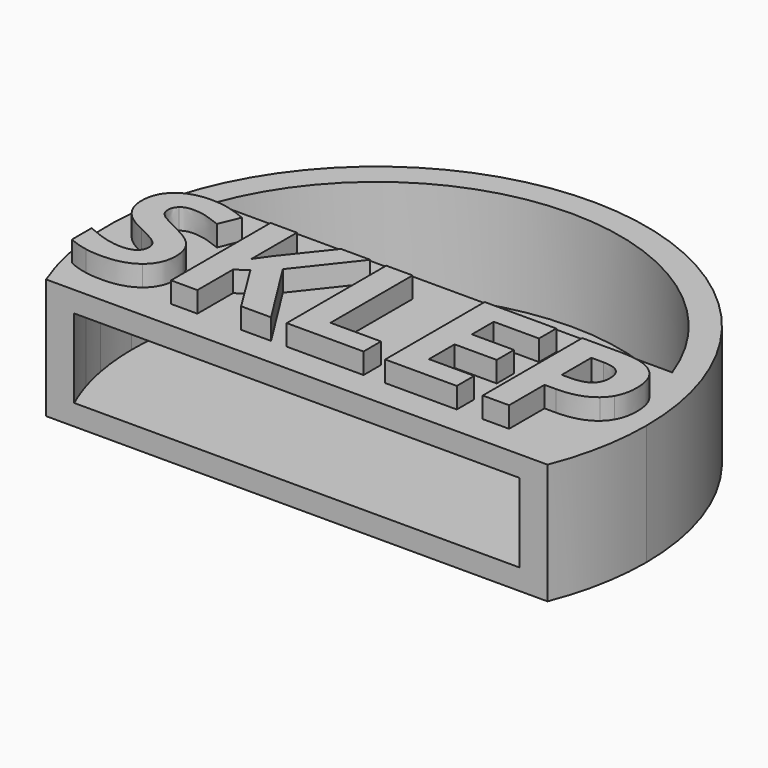
from build123d import *
from build123d import SkipClean  # not in build123d's __all__

# Parameters (mm, degrees)
F1_DEPTH = 5.8
F2_DEPTH = 6.8
F3_DEPTH = 4.8
F4_DEPTH = 1


with BuildPart() as f1:
    # F0 (on Top) → F1 (new body)
    with BuildSketch(Plane.XY):
        with BuildLine():
            ThreePointArc((-11.2352366102, -3.4397613744), (-11.0010890643, -4.1277765685), (-10.7248543114, -4.8))
            Line((-10.7248543114, -4.8), (10.7248543114, -4.8))
            ThreePointArc((10.7248543114, -4.8), (11.4520060458, -2.6294595504), (11.7445107181, -0.3591211385))
            add(Edge.make_bspline(
                [(11.7445107181, -0.3591211385), (11.6062328639, -0.5975122971), (11.3922086383, -0.7788061368)],
                knots=[0.6460850582, 0.6460850582, 0.6460850582, 1, 1, 1], degree=2))
            add(Edge.make_bspline(
                [(11.3922086383, -0.7788061368), (10.7874751266, -1.2910587101), (9.6724567211, -1.2910587101)],
                knots=[0, 0, 0, 1, 1, 1], degree=2))
            Line((9.6724567211, -1.2910587101), (9.1280653819, -1.2910587101))
            Line((9.1280653819, -1.2910587101), (9.1280653819, -3.4227115442))
            Line((9.1280653819, -3.4227115442), (7.8569443997, -3.4227115442))
            Line((7.8569443997, -3.4227115442), (7.8569443997, 2.570840332))
            Line((7.8569443997, 2.570840332), (9.7708406981, 2.570840332))
            add(Edge.make_bspline(
                [(9.7708406981, 2.570840332), (10.8622469491, 2.570840332), (11.4295945495, 2.1012208153)],
                knots=[0, 0, 0, 1, 1, 1], degree=2))
            add(Edge.make_bspline(
                [(11.4295945495, 2.1012208153), (11.5147201811, 2.0307584429), (11.5870734432, 1.9499305174)],
                knots=[0, 0, 0, 0.1500414058, 0.1500414058, 0.1500414058], degree=2))
            ThreePointArc((11.5870734432, 1.9499305174), (11.3639554223, 2.9871419718), (11.048189897, 4))
            Line((11.048189897, 4), (0, 4))
            Line((0, 4), (-11.048189897, 4))
            ThreePointArc((-11.048189897, 4), (-11.3300988619, 3.1130948875), (-11.5409335192, 2.2066611667))
            add(Edge.make_bspline(
                [(-11.5409335192, 2.2066611667), (-11.0025165801, 2.6561064453), (-10.0568101244, 2.6561064453)],
                knots=[0.0056134612, 0.0056134612, 0.0056134612, 1, 1, 1], degree=2))
            add(Edge.make_bspline(
                [(-10.0568101244, 2.6561064453), (-9.5898141805, 2.6561064453), (-9.1654512932, 2.5459163912)],
                knots=[0, 0, 0, 1, 1, 1], degree=2))
            add(Edge.make_bspline(
                [(-9.1654512932, 2.5459163912), (-8.7410884059, 2.435726337), (-8.278027821, 2.235023024)],
                knots=[0, 0, 0, 1, 1, 1], degree=2))
            Line((-8.278027821, 2.235023024), (-8.6873051652, 1.245936109))
            add(Edge.make_bspline(
                [(-8.6873051652, 1.245936109), (-9.1674189727, 1.4427040629), (-9.4809359126, 1.5207553513)],
                knots=[0, 0, 0, 1, 1, 1], degree=2))
            add(Edge.make_bspline(
                [(-9.4809359126, 1.5207553513), (-9.7944528525, 1.5988066397), (-10.0974755015, 1.5988066397)],
                knots=[0, 0, 0, 1, 1, 1], degree=2))
            add(Edge.make_bspline(
                [(-10.0974755015, 1.5988066397), (-10.4582167504, 1.5988066397), (-10.6510493452, 1.4308979857)],
                knots=[0, 0, 0, 1, 1, 1], degree=2))
            add(Edge.make_bspline(
                [(-10.6510493452, 1.4308979857), (-10.8438819401, 1.2629893317), (-10.8438819401, 0.9927613416)],
                knots=[0, 0, 0, 1, 1, 1], degree=2))
            add(Edge.make_bspline(
                [(-10.8438819401, 0.9927613416), (-10.8438819401, 0.8248526876), (-10.7658306517, 0.6995770903)],
                knots=[0, 0, 0, 1, 1, 1], degree=2))
            add(Edge.make_bspline(
                [(-10.7658306517, 0.6995770903), (-10.6877793633, 0.574301493), (-10.5179030297, 0.457552507)],
                knots=[0, 0, 0, 1, 1, 1], degree=2))
            add(Edge.make_bspline(
                [(-10.5179030297, 0.457552507), (-10.3480266962, 0.340803521), (-9.7131220982, 0.037780872)],
                knots=[0, 0, 0, 1, 1, 1], degree=2))
            add(Edge.make_bspline(
                [(-9.7131220982, 0.037780872), (-8.8722670419, -0.3649375404), (-8.5607177815, -0.7683118459)],
                knots=[0, 0, 0, 1, 1, 1], degree=2))
            add(Edge.make_bspline(
                [(-8.5607177815, -0.7683118459), (-8.2491685211, -1.1716861514), (-8.2491685211, -1.7580546541)],
                knots=[0, 0, 0, 1, 1, 1], degree=2))
            add(Edge.make_bspline(
                [(-8.2491685211, -1.7580546541), (-8.2491685211, -2.5700504105), (-8.8335693443, -3.0377022477)],
                knots=[0, 0, 0, 1, 1, 1], degree=2))
            add(Edge.make_bspline(
                [(-8.8335693443, -3.0377022477), (-9.4179701674, -3.5053540848), (-10.4582167504, -3.5053540848)],
                knots=[0, 0, 0, 1, 1, 1], degree=2))
            add(Edge.make_bspline(
                [(-10.4582167504, -3.5053540848), (-10.8669273339, -3.5053540848), (-11.2352366102, -3.4397613744)],
                knots=[0, 0, 0, 0.4256392724, 0.4256392724, 0.4256392724], degree=2))
        make_face()
        Polygon((-4.4489234379, -0.0815916867), (-2.3421945447, -3.4227115442), (-3.7851595401, -3.4227115442), (-5.3553678123, -0.8975228023), (-5.8918884333, -1.283187992), (-5.8918884333, -3.4227115442), (-7.1630094156, -3.4227115442), (-7.1630094156, 2.570840332), (-5.8918884333, 2.570840332), (-5.8918884333, -0.1721049455), (-5.3920978303, 0.5336361158), (-3.7681063174, 2.570840332), (-2.357935981, 2.570840332), align=None, mode=Mode.SUBTRACT)
        Polygon((2.1139437182, -3.4227115442), (-1.5879173881, -3.4227115442), (-1.5879173881, 2.570840332), (-0.3167964058, 2.570840332), (-0.3167964058, -2.3732824566), (2.1139437182, -2.3732824566), align=None, mode=Mode.SUBTRACT)
        Polygon((6.6068119992, -2.3732824566), (6.6068119992, -3.4227115442), (3.1555020876, -3.4227115442), (3.1555020876, 2.570840332), (6.6068119992, 2.570840332), (6.6068119992, 1.5292819626), (4.4266230698, 1.5292819626), (4.4266230698, 0.2135602441), (6.4559565678, 0.2135602441), (6.4559565678, -0.8279981252), (4.4266230698, -0.8279981252), (4.4266230698, -2.3732824566), align=None, mode=Mode.SUBTRACT)
        with BuildLine():
            ThreePointArc((12.0813906484, -4.8), (12.7682825476, -2.4435549483), (13, 0))
            ThreePointArc((13, 0), (-2.4435549483, 12.7682825476), (-12.0813906484, -4.8))
            Line((-12.0813906484, -4.8), (-10.7248543114, -4.8))
            ThreePointArc((-10.7248543114, -4.8), (-11.0010890643, -4.1277765685), (-11.2352366102, -3.4397613744))
            add(Edge.make_bspline(
                [(-11.2352366102, -3.4397613744), (-11.7322358244, -3.3512500943), (-12.1556682995, -3.1433010496)],
                knots=[0.4256392724, 0.4256392724, 0.4256392724, 1, 1, 1], degree=2))
            Line((-12.1556682995, -3.1433010496), (-12.1556682995, -1.9626933261))
            add(Edge.make_bspline(
                [(-12.1556682995, -1.9626933261), (-11.8188714135, -2.113595827), (-11.5393997189, -2.2146679495)],
                knots=[0, 0, 0, 0.5557288985, 0.5557288985, 0.5557288985], degree=2))
            ThreePointArc((-11.5393997189, -2.2146679495), (-11.6944490524, -1.1412104809), (-11.749856705, -0.0580294135))
            add(Edge.make_bspline(
                [(-11.749856705, -0.0580294135), (-11.8475051096, 0.069605704), (-11.9221703275, 0.2135602441)],
                knots=[0.5446501339, 0.5446501339, 0.5446501339, 1, 1, 1], degree=2))
            add(Edge.make_bspline(
                [(-11.9221703275, 0.2135602441), (-12.0861436224, 0.5297007567), (-12.0861436224, 0.9507841781)],
                knots=[0, 0, 0, 1, 1, 1], degree=2))
            add(Edge.make_bspline(
                [(-12.0861436224, 0.9507841781), (-12.0861436224, 1.7470384983), (-11.5469994287, 2.2015724718)],
                knots=[0, 0, 0, 1, 1, 1], degree=2))
            add(Edge.make_bspline(
                [(-11.5469994287, 2.2015724718), (-11.5439729637, 2.2041239807), (-11.5409335192, 2.2066611667)],
                knots=[0, 0, 0, 0.0056134612, 0.0056134612, 0.0056134612], degree=2))
            ThreePointArc((-11.5409335192, 2.2066611667), (-11.3300988619, 3.1130948875), (-11.048189897, 4))
            ThreePointArc((-11.048189897, 4), (0, 11.75), (11.048189897, 4))
            ThreePointArc((11.048189897, 4), (11.3639554223, 2.9871419718), (11.5870734432, 1.9499305174))
            add(Edge.make_bspline(
                [(11.5870734432, 1.9499305174), (11.99694215, 1.4920543096), (11.99694215, 0.7015447698)],
                knots=[0.1500414058, 0.1500414058, 0.1500414058, 1, 1, 1], degree=2))
            add(Edge.make_bspline(
                [(11.99694215, 0.7015447698), (11.99694215, 0.0760709018), (11.7445107181, -0.3591211385)],
                knots=[0, 0, 0, 0.6460850582, 0.6460850582, 0.6460850582], degree=2))
            ThreePointArc((11.7445107181, -0.3591211385), (11.4520060458, -2.6294595504), (10.7248543114, -4.8))
            Line((10.7248543114, -4.8), (12.0813906484, -4.8))
        make_face()
        with BuildLine():
            ThreePointArc((-11.749856705, -0.0580294135), (-11.6944490524, -1.1412104809), (-11.5393997189, -2.2146679495))
            add(Edge.make_bspline(
                [(-11.5393997189, -2.2146679495), (-11.3159792743, -2.2954689), (-11.1291954732, -2.3444231567)],
                knots=[0.5557288985, 0.5557288985, 0.5557288985, 1, 1, 1], degree=2))
            add(Edge.make_bspline(
                [(-11.1291954732, -2.3444231567), (-10.708767945, -2.4546132109), (-10.3598327734, -2.4546132109)],
                knots=[0, 0, 0, 1, 1, 1], degree=2))
            add(Edge.make_bspline(
                [(-10.3598327734, -2.4546132109), (-9.9426847111, -2.4546132109), (-9.7190251369, -2.2952311682)],
                knots=[0, 0, 0, 1, 1, 1], degree=2))
            add(Edge.make_bspline(
                [(-9.7190251369, -2.2952311682), (-9.4953655626, -2.1358491256), (-9.4953655626, -1.819708613)],
                knots=[0, 0, 0, 1, 1, 1], degree=2))
            add(Edge.make_bspline(
                [(-9.4953655626, -1.819708613), (-9.4953655626, -1.6439292408), (-9.5937495395, -1.5061916731)],
                knots=[0, 0, 0, 1, 1, 1], degree=2))
            add(Edge.make_bspline(
                [(-9.5937495395, -1.5061916731), (-9.6921335165, -1.3684541053), (-9.8829984318, -1.2418667216)],
                knots=[0, 0, 0, 1, 1, 1], degree=2))
            add(Edge.make_bspline(
                [(-9.8829984318, -1.2418667216), (-10.0738633471, -1.115279338), (-10.6602318497, -0.8358688434)],
                knots=[0, 0, 0, 1, 1, 1], degree=2))
            add(Edge.make_bspline(
                [(-10.6602318497, -0.8358688434), (-11.208558548, -0.5774469306), (-11.4833777903, -0.3400135995)],
                knots=[0, 0, 0, 1, 1, 1], degree=2))
            add(Edge.make_bspline(
                [(-11.4833777903, -0.3400135995), (-11.6330581274, -0.210695504), (-11.749856705, -0.0580294135)],
                knots=[0, 0, 0, 0.5446501339, 0.5446501339, 0.5446501339], degree=2))
        make_face()
    extrude(amount=F1_DEPTH)



with BuildPart() as f1b:
    # F0 (on Top) → F1, piece 2 (new body)
    with BuildSketch(Plane.XY):
        with BuildLine():
            Line((9.1280653819, 1.5292819626), (9.1280653819, -0.2495003407))
            Line((9.1280653819, -0.2495003407), (9.5465252306, -0.2495003407))
            add(Edge.make_bspline(
                [(9.5465252306, -0.2495003407), (10.1315819469, -0.2495003407), (10.4227985187, -0.0179700483)],
                knots=[0, 0, 0, 1, 1, 1], degree=2))
            add(Edge.make_bspline(
                [(10.4227985187, -0.0179700483), (10.7140150905, 0.2135602441), (10.7140150905, 0.6556322472)],
                knots=[0, 0, 0, 1, 1, 1], degree=2))
            add(Edge.make_bspline(
                [(10.7140150905, 0.6556322472), (10.7140150905, 1.1029513958), (10.4700228276, 1.3161166792)],
                knots=[0, 0, 0, 1, 1, 1], degree=2))
            add(Edge.make_bspline(
                [(10.4700228276, 1.3161166792), (10.2260305648, 1.5292819626), (9.7052513801, 1.5292819626)],
                knots=[0, 0, 0, 1, 1, 1], degree=2))
            Line((9.7052513801, 1.5292819626), (9.1280653819, 1.5292819626))
        make_face()
    extrude(amount=F1_DEPTH)


with BuildPart() as f1_1:
    add(f1.part, clean=False)

    add(f1b.part)  # F2 merges F1b
    # F0 (on Top) → F2 (join)
    with BuildSketch(Plane.XY):
        Polygon((-1.5879173881, 2.570840332), (-1.5879173881, -3.4227115442), (2.1139437182, -3.4227115442), (2.1139437182, -2.3732824566), (-0.3167964058, -2.3732824566), (-0.3167964058, 2.570840332), align=None)
        Polygon((3.1555020876, -3.4227115442), (6.6068119992, -3.4227115442), (6.6068119992, -2.3732824566), (4.4266230698, -2.3732824566), (4.4266230698, -0.8279981252), (6.4559565678, -0.8279981252), (6.4559565678, 0.2135602441), (4.4266230698, 0.2135602441), (4.4266230698, 1.5292819626), (6.6068119992, 1.5292819626), (6.6068119992, 2.570840332), (3.1555020876, 2.570840332), align=None)
        with BuildLine():
            add(Edge.make_bspline(
                [(11.7445107181, -0.3591211385), (11.6062328639, -0.5975122971), (11.3922086383, -0.7788061368)],
                knots=[0.6460850582, 0.6460850582, 0.6460850582, 1, 1, 1], degree=2))
            ThreePointArc((11.7445107181, -0.3591211385), (11.7486275994, -0.1795815444), (11.75, 0))
            ThreePointArc((11.75, 0), (11.7091975164, 0.9783626738), (11.5870734432, 1.9499305174))
            add(Edge.make_bspline(
                [(11.4295945495, 2.1012208153), (11.5147201811, 2.0307584429), (11.5870734432, 1.9499305174)],
                knots=[0, 0, 0, 0.1500414058, 0.1500414058, 0.1500414058], degree=2))
            add(Edge.make_bspline(
                [(9.7708406981, 2.570840332), (10.8622469491, 2.570840332), (11.4295945495, 2.1012208153)],
                knots=[0, 0, 0, 1, 1, 1], degree=2))
            Line((9.7708406981, 2.570840332), (7.8569443997, 2.570840332))
            Line((7.8569443997, 2.570840332), (7.8569443997, -3.4227115442))
            Line((7.8569443997, -3.4227115442), (9.1280653819, -3.4227115442))
            Line((9.1280653819, -3.4227115442), (9.1280653819, -1.2910587101))
            Line((9.1280653819, -1.2910587101), (9.6724567211, -1.2910587101))
            add(Edge.make_bspline(
                [(11.3922086383, -0.7788061368), (10.7874751266, -1.2910587101), (9.6724567211, -1.2910587101)],
                knots=[0, 0, 0, 1, 1, 1], degree=2))
        make_face()
        with BuildLine():
            Line((9.5465252306, -0.2495003407), (9.1280653819, -0.2495003407))
            Line((9.1280653819, -0.2495003407), (9.1280653819, 1.5292819626))
            Line((9.1280653819, 1.5292819626), (9.7052513801, 1.5292819626))
            add(Edge.make_bspline(
                [(10.4700228276, 1.3161166792), (10.2260305648, 1.5292819626), (9.7052513801, 1.5292819626)],
                knots=[0, 0, 0, 1, 1, 1], degree=2))
            add(Edge.make_bspline(
                [(10.7140150905, 0.6556322472), (10.7140150905, 1.1029513958), (10.4700228276, 1.3161166792)],
                knots=[0, 0, 0, 1, 1, 1], degree=2))
            add(Edge.make_bspline(
                [(10.4227985187, -0.0179700483), (10.7140150905, 0.2135602441), (10.7140150905, 0.6556322472)],
                knots=[0, 0, 0, 1, 1, 1], degree=2))
            add(Edge.make_bspline(
                [(9.5465252306, -0.2495003407), (10.1315819469, -0.2495003407), (10.4227985187, -0.0179700483)],
                knots=[0, 0, 0, 1, 1, 1], degree=2))
        make_face(mode=Mode.SUBTRACT)
        Polygon((-3.7851595401, -3.4227115442), (-2.3421945447, -3.4227115442), (-4.4489234379, -0.0815916867), (-2.357935981, 2.570840332), (-3.7681063174, 2.570840332), (-5.3920978303, 0.5336361158), (-5.8918884333, -0.1721049455), (-5.8918884333, 2.570840332), (-7.1630094156, 2.570840332), (-7.1630094156, -3.4227115442), (-5.8918884333, -3.4227115442), (-5.8918884333, -1.283187992), (-5.3553678123, -0.8975228023), align=None)
        with BuildLine():
            ThreePointArc((-11.5393997189, -2.2146679495), (-11.4037813227, -2.8313020934), (-11.2352366102, -3.4397613744))
            add(Edge.make_bspline(
                [(-10.4582167504, -3.5053540848), (-10.8669273339, -3.5053540848), (-11.2352366102, -3.4397613744)],
                knots=[0, 0, 0, 0.4256392724, 0.4256392724, 0.4256392724], degree=2))
            add(Edge.make_bspline(
                [(-8.8335693443, -3.0377022477), (-9.4179701674, -3.5053540848), (-10.4582167504, -3.5053540848)],
                knots=[0, 0, 0, 1, 1, 1], degree=2))
            add(Edge.make_bspline(
                [(-8.2491685211, -1.7580546541), (-8.2491685211, -2.5700504105), (-8.8335693443, -3.0377022477)],
                knots=[0, 0, 0, 1, 1, 1], degree=2))
            add(Edge.make_bspline(
                [(-8.5607177815, -0.7683118459), (-8.2491685211, -1.1716861514), (-8.2491685211, -1.7580546541)],
                knots=[0, 0, 0, 1, 1, 1], degree=2))
            add(Edge.make_bspline(
                [(-9.7131220982, 0.037780872), (-8.8722670419, -0.3649375404), (-8.5607177815, -0.7683118459)],
                knots=[0, 0, 0, 1, 1, 1], degree=2))
            add(Edge.make_bspline(
                [(-10.5179030297, 0.457552507), (-10.3480266962, 0.340803521), (-9.7131220982, 0.037780872)],
                knots=[0, 0, 0, 1, 1, 1], degree=2))
            add(Edge.make_bspline(
                [(-10.7658306517, 0.6995770903), (-10.6877793633, 0.574301493), (-10.5179030297, 0.457552507)],
                knots=[0, 0, 0, 1, 1, 1], degree=2))
            add(Edge.make_bspline(
                [(-10.8438819401, 0.9927613416), (-10.8438819401, 0.8248526876), (-10.7658306517, 0.6995770903)],
                knots=[0, 0, 0, 1, 1, 1], degree=2))
            add(Edge.make_bspline(
                [(-10.6510493452, 1.4308979857), (-10.8438819401, 1.2629893317), (-10.8438819401, 0.9927613416)],
                knots=[0, 0, 0, 1, 1, 1], degree=2))
            add(Edge.make_bspline(
                [(-10.0974755015, 1.5988066397), (-10.4582167504, 1.5988066397), (-10.6510493452, 1.4308979857)],
                knots=[0, 0, 0, 1, 1, 1], degree=2))
            add(Edge.make_bspline(
                [(-9.4809359126, 1.5207553513), (-9.7944528525, 1.5988066397), (-10.0974755015, 1.5988066397)],
                knots=[0, 0, 0, 1, 1, 1], degree=2))
            add(Edge.make_bspline(
                [(-8.6873051652, 1.245936109), (-9.1674189727, 1.4427040629), (-9.4809359126, 1.5207553513)],
                knots=[0, 0, 0, 1, 1, 1], degree=2))
            Line((-8.6873051652, 1.245936109), (-8.278027821, 2.235023024))
            add(Edge.make_bspline(
                [(-9.1654512932, 2.5459163912), (-8.7410884059, 2.435726337), (-8.278027821, 2.235023024)],
                knots=[0, 0, 0, 1, 1, 1], degree=2))
            add(Edge.make_bspline(
                [(-10.0568101244, 2.6561064453), (-9.5898141805, 2.6561064453), (-9.1654512932, 2.5459163912)],
                knots=[0, 0, 0, 1, 1, 1], degree=2))
            add(Edge.make_bspline(
                [(-11.5409335192, 2.2066611667), (-11.0025165801, 2.6561064453), (-10.0568101244, 2.6561064453)],
                knots=[0.0056134612, 0.0056134612, 0.0056134612, 1, 1, 1], degree=2))
            ThreePointArc((-11.5409335192, 2.2066611667), (-11.7003176526, 1.0793826139), (-11.749856705, -0.0580294135))
            add(Edge.make_bspline(
                [(-11.4833777903, -0.3400135995), (-11.6330581274, -0.210695504), (-11.749856705, -0.0580294135)],
                knots=[0, 0, 0, 0.5446501339, 0.5446501339, 0.5446501339], degree=2))
            add(Edge.make_bspline(
                [(-10.6602318497, -0.8358688434), (-11.208558548, -0.5774469306), (-11.4833777903, -0.3400135995)],
                knots=[0, 0, 0, 1, 1, 1], degree=2))
            add(Edge.make_bspline(
                [(-9.8829984318, -1.2418667216), (-10.0738633471, -1.115279338), (-10.6602318497, -0.8358688434)],
                knots=[0, 0, 0, 1, 1, 1], degree=2))
            add(Edge.make_bspline(
                [(-9.5937495395, -1.5061916731), (-9.6921335165, -1.3684541053), (-9.8829984318, -1.2418667216)],
                knots=[0, 0, 0, 1, 1, 1], degree=2))
            add(Edge.make_bspline(
                [(-9.4953655626, -1.819708613), (-9.4953655626, -1.6439292408), (-9.5937495395, -1.5061916731)],
                knots=[0, 0, 0, 1, 1, 1], degree=2))
            add(Edge.make_bspline(
                [(-9.7190251369, -2.2952311682), (-9.4953655626, -2.1358491256), (-9.4953655626, -1.819708613)],
                knots=[0, 0, 0, 1, 1, 1], degree=2))
            add(Edge.make_bspline(
                [(-10.3598327734, -2.4546132109), (-9.9426847111, -2.4546132109), (-9.7190251369, -2.2952311682)],
                knots=[0, 0, 0, 1, 1, 1], degree=2))
            add(Edge.make_bspline(
                [(-11.1291954732, -2.3444231567), (-10.708767945, -2.4546132109), (-10.3598327734, -2.4546132109)],
                knots=[0, 0, 0, 1, 1, 1], degree=2))
            add(Edge.make_bspline(
                [(-11.5393997189, -2.2146679495), (-11.3159792743, -2.2954689), (-11.1291954732, -2.3444231567)],
                knots=[0.5557288985, 0.5557288985, 0.5557288985, 1, 1, 1], degree=2))
        make_face()
        with BuildLine():
            add(Edge.make_bspline(
                [(-11.2352366102, -3.4397613744), (-11.7322358244, -3.3512500943), (-12.1556682995, -3.1433010496)],
                knots=[0.4256392724, 0.4256392724, 0.4256392724, 1, 1, 1], degree=2))
            ThreePointArc((-11.2352366102, -3.4397613744), (-11.4037813227, -2.8313020934), (-11.5393997189, -2.2146679495))
            add(Edge.make_bspline(
                [(-12.1556682995, -1.9626933261), (-11.8188714135, -2.113595827), (-11.5393997189, -2.2146679495)],
                knots=[0, 0, 0, 0.5557288985, 0.5557288985, 0.5557288985], degree=2))
            Line((-12.1556682995, -1.9626933261), (-12.1556682995, -3.1433010496))
        make_face()
        with BuildLine():
            add(Edge.make_bspline(
                [(-11.749856705, -0.0580294135), (-11.8475051096, 0.069605704), (-11.9221703275, 0.2135602441)],
                knots=[0.5446501339, 0.5446501339, 0.5446501339, 1, 1, 1], degree=2))
            ThreePointArc((-11.749856705, -0.0580294135), (-11.7003176526, 1.0793826139), (-11.5409335192, 2.2066611667))
            add(Edge.make_bspline(
                [(-11.5469994287, 2.2015724718), (-11.5439729637, 2.2041239807), (-11.5409335192, 2.2066611667)],
                knots=[0, 0, 0, 0.0056134612, 0.0056134612, 0.0056134612], degree=2))
            add(Edge.make_bspline(
                [(-12.0861436224, 0.9507841781), (-12.0861436224, 1.7470384983), (-11.5469994287, 2.2015724718)],
                knots=[0, 0, 0, 1, 1, 1], degree=2))
            add(Edge.make_bspline(
                [(-11.9221703275, 0.2135602441), (-12.0861436224, 0.5297007567), (-12.0861436224, 0.9507841781)],
                knots=[0, 0, 0, 1, 1, 1], degree=2))
        make_face()
        with BuildLine():
            ThreePointArc((11.75, 0), (11.7486275994, -0.1795815444), (11.7445107181, -0.3591211385))
            add(Edge.make_bspline(
                [(11.99694215, 0.7015447698), (11.99694215, 0.0760709018), (11.7445107181, -0.3591211385)],
                knots=[0, 0, 0, 0.6460850582, 0.6460850582, 0.6460850582], degree=2))
            add(Edge.make_bspline(
                [(11.5870734432, 1.9499305174), (11.99694215, 1.4920543096), (11.99694215, 0.7015447698)],
                knots=[0.1500414058, 0.1500414058, 0.1500414058, 1, 1, 1], degree=2))
            ThreePointArc((11.5870734432, 1.9499305174), (11.7091975164, 0.9783626738), (11.75, 0))
        make_face()
    extrude(amount=F2_DEPTH)

    # F0 (on Top) → F3 (cut)
    with BuildSketch(Plane.XY):
        with BuildLine():
            ThreePointArc((-11.2352366102, -3.4397613744), (-11.0010890643, -4.1277765685), (-10.7248543114, -4.8))
            Line((-10.7248543114, -4.8), (10.7248543114, -4.8))
            ThreePointArc((10.7248543114, -4.8), (11.4520060458, -2.6294595504), (11.7445107181, -0.3591211385))
            add(Edge.make_bspline(
                [(11.7445107181, -0.3591211385), (11.6062328639, -0.5975122971), (11.3922086383, -0.7788061368)],
                knots=[0.6460850582, 0.6460850582, 0.6460850582, 1, 1, 1], degree=2))
            add(Edge.make_bspline(
                [(11.3922086383, -0.7788061368), (10.7874751266, -1.2910587101), (9.6724567211, -1.2910587101)],
                knots=[0, 0, 0, 1, 1, 1], degree=2))
            Line((9.6724567211, -1.2910587101), (9.1280653819, -1.2910587101))
            Line((9.1280653819, -1.2910587101), (9.1280653819, -3.4227115442))
            Line((9.1280653819, -3.4227115442), (7.8569443997, -3.4227115442))
            Line((7.8569443997, -3.4227115442), (7.8569443997, 2.570840332))
            Line((7.8569443997, 2.570840332), (9.7708406981, 2.570840332))
            add(Edge.make_bspline(
                [(9.7708406981, 2.570840332), (10.8622469491, 2.570840332), (11.4295945495, 2.1012208153)],
                knots=[0, 0, 0, 1, 1, 1], degree=2))
            add(Edge.make_bspline(
                [(11.4295945495, 2.1012208153), (11.5147201811, 2.0307584429), (11.5870734432, 1.9499305174)],
                knots=[0, 0, 0, 0.1500414058, 0.1500414058, 0.1500414058], degree=2))
            ThreePointArc((11.5870734432, 1.9499305174), (11.3639554223, 2.9871419718), (11.048189897, 4))
            Line((11.048189897, 4), (0, 4))
            Line((0, 4), (-11.048189897, 4))
            ThreePointArc((-11.048189897, 4), (-11.3300988619, 3.1130948875), (-11.5409335192, 2.2066611667))
            add(Edge.make_bspline(
                [(-11.5409335192, 2.2066611667), (-11.0025165801, 2.6561064453), (-10.0568101244, 2.6561064453)],
                knots=[0.0056134612, 0.0056134612, 0.0056134612, 1, 1, 1], degree=2))
            add(Edge.make_bspline(
                [(-10.0568101244, 2.6561064453), (-9.5898141805, 2.6561064453), (-9.1654512932, 2.5459163912)],
                knots=[0, 0, 0, 1, 1, 1], degree=2))
            add(Edge.make_bspline(
                [(-9.1654512932, 2.5459163912), (-8.7410884059, 2.435726337), (-8.278027821, 2.235023024)],
                knots=[0, 0, 0, 1, 1, 1], degree=2))
            Line((-8.278027821, 2.235023024), (-8.6873051652, 1.245936109))
            add(Edge.make_bspline(
                [(-8.6873051652, 1.245936109), (-9.1674189727, 1.4427040629), (-9.4809359126, 1.5207553513)],
                knots=[0, 0, 0, 1, 1, 1], degree=2))
            add(Edge.make_bspline(
                [(-9.4809359126, 1.5207553513), (-9.7944528525, 1.5988066397), (-10.0974755015, 1.5988066397)],
                knots=[0, 0, 0, 1, 1, 1], degree=2))
            add(Edge.make_bspline(
                [(-10.0974755015, 1.5988066397), (-10.4582167504, 1.5988066397), (-10.6510493452, 1.4308979857)],
                knots=[0, 0, 0, 1, 1, 1], degree=2))
            add(Edge.make_bspline(
                [(-10.6510493452, 1.4308979857), (-10.8438819401, 1.2629893317), (-10.8438819401, 0.9927613416)],
                knots=[0, 0, 0, 1, 1, 1], degree=2))
            add(Edge.make_bspline(
                [(-10.8438819401, 0.9927613416), (-10.8438819401, 0.8248526876), (-10.7658306517, 0.6995770903)],
                knots=[0, 0, 0, 1, 1, 1], degree=2))
            add(Edge.make_bspline(
                [(-10.7658306517, 0.6995770903), (-10.6877793633, 0.574301493), (-10.5179030297, 0.457552507)],
                knots=[0, 0, 0, 1, 1, 1], degree=2))
            add(Edge.make_bspline(
                [(-10.5179030297, 0.457552507), (-10.3480266962, 0.340803521), (-9.7131220982, 0.037780872)],
                knots=[0, 0, 0, 1, 1, 1], degree=2))
            add(Edge.make_bspline(
                [(-9.7131220982, 0.037780872), (-8.8722670419, -0.3649375404), (-8.5607177815, -0.7683118459)],
                knots=[0, 0, 0, 1, 1, 1], degree=2))
            add(Edge.make_bspline(
                [(-8.5607177815, -0.7683118459), (-8.2491685211, -1.1716861514), (-8.2491685211, -1.7580546541)],
                knots=[0, 0, 0, 1, 1, 1], degree=2))
            add(Edge.make_bspline(
                [(-8.2491685211, -1.7580546541), (-8.2491685211, -2.5700504105), (-8.8335693443, -3.0377022477)],
                knots=[0, 0, 0, 1, 1, 1], degree=2))
            add(Edge.make_bspline(
                [(-8.8335693443, -3.0377022477), (-9.4179701674, -3.5053540848), (-10.4582167504, -3.5053540848)],
                knots=[0, 0, 0, 1, 1, 1], degree=2))
            add(Edge.make_bspline(
                [(-10.4582167504, -3.5053540848), (-10.8669273339, -3.5053540848), (-11.2352366102, -3.4397613744)],
                knots=[0, 0, 0, 0.4256392724, 0.4256392724, 0.4256392724], degree=2))
        make_face()
        Polygon((-4.4489234379, -0.0815916867), (-2.3421945447, -3.4227115442), (-3.7851595401, -3.4227115442), (-5.3553678123, -0.8975228023), (-5.8918884333, -1.283187992), (-5.8918884333, -3.4227115442), (-7.1630094156, -3.4227115442), (-7.1630094156, 2.570840332), (-5.8918884333, 2.570840332), (-5.8918884333, -0.1721049455), (-5.3920978303, 0.5336361158), (-3.7681063174, 2.570840332), (-2.357935981, 2.570840332), align=None, mode=Mode.SUBTRACT)
        Polygon((2.1139437182, -3.4227115442), (-1.5879173881, -3.4227115442), (-1.5879173881, 2.570840332), (-0.3167964058, 2.570840332), (-0.3167964058, -2.3732824566), (2.1139437182, -2.3732824566), align=None, mode=Mode.SUBTRACT)
        Polygon((6.6068119992, -2.3732824566), (6.6068119992, -3.4227115442), (3.1555020876, -3.4227115442), (3.1555020876, 2.570840332), (6.6068119992, 2.570840332), (6.6068119992, 1.5292819626), (4.4266230698, 1.5292819626), (4.4266230698, 0.2135602441), (6.4559565678, 0.2135602441), (6.4559565678, -0.8279981252), (4.4266230698, -0.8279981252), (4.4266230698, -2.3732824566), align=None, mode=Mode.SUBTRACT)
        with BuildLine():
            ThreePointArc((-11.5393997189, -2.2146679495), (-11.4037813227, -2.8313020934), (-11.2352366102, -3.4397613744))
            add(Edge.make_bspline(
                [(-10.4582167504, -3.5053540848), (-10.8669273339, -3.5053540848), (-11.2352366102, -3.4397613744)],
                knots=[0, 0, 0, 0.4256392724, 0.4256392724, 0.4256392724], degree=2))
            add(Edge.make_bspline(
                [(-8.8335693443, -3.0377022477), (-9.4179701674, -3.5053540848), (-10.4582167504, -3.5053540848)],
                knots=[0, 0, 0, 1, 1, 1], degree=2))
            add(Edge.make_bspline(
                [(-8.2491685211, -1.7580546541), (-8.2491685211, -2.5700504105), (-8.8335693443, -3.0377022477)],
                knots=[0, 0, 0, 1, 1, 1], degree=2))
            add(Edge.make_bspline(
                [(-8.5607177815, -0.7683118459), (-8.2491685211, -1.1716861514), (-8.2491685211, -1.7580546541)],
                knots=[0, 0, 0, 1, 1, 1], degree=2))
            add(Edge.make_bspline(
                [(-9.7131220982, 0.037780872), (-8.8722670419, -0.3649375404), (-8.5607177815, -0.7683118459)],
                knots=[0, 0, 0, 1, 1, 1], degree=2))
            add(Edge.make_bspline(
                [(-10.5179030297, 0.457552507), (-10.3480266962, 0.340803521), (-9.7131220982, 0.037780872)],
                knots=[0, 0, 0, 1, 1, 1], degree=2))
            add(Edge.make_bspline(
                [(-10.7658306517, 0.6995770903), (-10.6877793633, 0.574301493), (-10.5179030297, 0.457552507)],
                knots=[0, 0, 0, 1, 1, 1], degree=2))
            add(Edge.make_bspline(
                [(-10.8438819401, 0.9927613416), (-10.8438819401, 0.8248526876), (-10.7658306517, 0.6995770903)],
                knots=[0, 0, 0, 1, 1, 1], degree=2))
            add(Edge.make_bspline(
                [(-10.6510493452, 1.4308979857), (-10.8438819401, 1.2629893317), (-10.8438819401, 0.9927613416)],
                knots=[0, 0, 0, 1, 1, 1], degree=2))
            add(Edge.make_bspline(
                [(-10.0974755015, 1.5988066397), (-10.4582167504, 1.5988066397), (-10.6510493452, 1.4308979857)],
                knots=[0, 0, 0, 1, 1, 1], degree=2))
            add(Edge.make_bspline(
                [(-9.4809359126, 1.5207553513), (-9.7944528525, 1.5988066397), (-10.0974755015, 1.5988066397)],
                knots=[0, 0, 0, 1, 1, 1], degree=2))
            add(Edge.make_bspline(
                [(-8.6873051652, 1.245936109), (-9.1674189727, 1.4427040629), (-9.4809359126, 1.5207553513)],
                knots=[0, 0, 0, 1, 1, 1], degree=2))
            Line((-8.6873051652, 1.245936109), (-8.278027821, 2.235023024))
            add(Edge.make_bspline(
                [(-9.1654512932, 2.5459163912), (-8.7410884059, 2.435726337), (-8.278027821, 2.235023024)],
                knots=[0, 0, 0, 1, 1, 1], degree=2))
            add(Edge.make_bspline(
                [(-10.0568101244, 2.6561064453), (-9.5898141805, 2.6561064453), (-9.1654512932, 2.5459163912)],
                knots=[0, 0, 0, 1, 1, 1], degree=2))
            add(Edge.make_bspline(
                [(-11.5409335192, 2.2066611667), (-11.0025165801, 2.6561064453), (-10.0568101244, 2.6561064453)],
                knots=[0.0056134612, 0.0056134612, 0.0056134612, 1, 1, 1], degree=2))
            ThreePointArc((-11.5409335192, 2.2066611667), (-11.7003176526, 1.0793826139), (-11.749856705, -0.0580294135))
            add(Edge.make_bspline(
                [(-11.4833777903, -0.3400135995), (-11.6330581274, -0.210695504), (-11.749856705, -0.0580294135)],
                knots=[0, 0, 0, 0.5446501339, 0.5446501339, 0.5446501339], degree=2))
            add(Edge.make_bspline(
                [(-10.6602318497, -0.8358688434), (-11.208558548, -0.5774469306), (-11.4833777903, -0.3400135995)],
                knots=[0, 0, 0, 1, 1, 1], degree=2))
            add(Edge.make_bspline(
                [(-9.8829984318, -1.2418667216), (-10.0738633471, -1.115279338), (-10.6602318497, -0.8358688434)],
                knots=[0, 0, 0, 1, 1, 1], degree=2))
            add(Edge.make_bspline(
                [(-9.5937495395, -1.5061916731), (-9.6921335165, -1.3684541053), (-9.8829984318, -1.2418667216)],
                knots=[0, 0, 0, 1, 1, 1], degree=2))
            add(Edge.make_bspline(
                [(-9.4953655626, -1.819708613), (-9.4953655626, -1.6439292408), (-9.5937495395, -1.5061916731)],
                knots=[0, 0, 0, 1, 1, 1], degree=2))
            add(Edge.make_bspline(
                [(-9.7190251369, -2.2952311682), (-9.4953655626, -2.1358491256), (-9.4953655626, -1.819708613)],
                knots=[0, 0, 0, 1, 1, 1], degree=2))
            add(Edge.make_bspline(
                [(-10.3598327734, -2.4546132109), (-9.9426847111, -2.4546132109), (-9.7190251369, -2.2952311682)],
                knots=[0, 0, 0, 1, 1, 1], degree=2))
            add(Edge.make_bspline(
                [(-11.1291954732, -2.3444231567), (-10.708767945, -2.4546132109), (-10.3598327734, -2.4546132109)],
                knots=[0, 0, 0, 1, 1, 1], degree=2))
            add(Edge.make_bspline(
                [(-11.5393997189, -2.2146679495), (-11.3159792743, -2.2954689), (-11.1291954732, -2.3444231567)],
                knots=[0.5557288985, 0.5557288985, 0.5557288985, 1, 1, 1], degree=2))
        make_face()
        Polygon((-3.7851595401, -3.4227115442), (-2.3421945447, -3.4227115442), (-4.4489234379, -0.0815916867), (-2.357935981, 2.570840332), (-3.7681063174, 2.570840332), (-5.3920978303, 0.5336361158), (-5.8918884333, -0.1721049455), (-5.8918884333, 2.570840332), (-7.1630094156, 2.570840332), (-7.1630094156, -3.4227115442), (-5.8918884333, -3.4227115442), (-5.8918884333, -1.283187992), (-5.3553678123, -0.8975228023), align=None)
        Polygon((-1.5879173881, 2.570840332), (-1.5879173881, -3.4227115442), (2.1139437182, -3.4227115442), (2.1139437182, -2.3732824566), (-0.3167964058, -2.3732824566), (-0.3167964058, 2.570840332), align=None)
        Polygon((3.1555020876, -3.4227115442), (6.6068119992, -3.4227115442), (6.6068119992, -2.3732824566), (4.4266230698, -2.3732824566), (4.4266230698, -0.8279981252), (6.4559565678, -0.8279981252), (6.4559565678, 0.2135602441), (4.4266230698, 0.2135602441), (4.4266230698, 1.5292819626), (6.6068119992, 1.5292819626), (6.6068119992, 2.570840332), (3.1555020876, 2.570840332), align=None)
        with BuildLine():
            add(Edge.make_bspline(
                [(11.7445107181, -0.3591211385), (11.6062328639, -0.5975122971), (11.3922086383, -0.7788061368)],
                knots=[0.6460850582, 0.6460850582, 0.6460850582, 1, 1, 1], degree=2))
            ThreePointArc((11.7445107181, -0.3591211385), (11.7486275994, -0.1795815444), (11.75, 0))
            ThreePointArc((11.75, 0), (11.7091975164, 0.9783626738), (11.5870734432, 1.9499305174))
            add(Edge.make_bspline(
                [(11.4295945495, 2.1012208153), (11.5147201811, 2.0307584429), (11.5870734432, 1.9499305174)],
                knots=[0, 0, 0, 0.1500414058, 0.1500414058, 0.1500414058], degree=2))
            add(Edge.make_bspline(
                [(9.7708406981, 2.570840332), (10.8622469491, 2.570840332), (11.4295945495, 2.1012208153)],
                knots=[0, 0, 0, 1, 1, 1], degree=2))
            Line((9.7708406981, 2.570840332), (7.8569443997, 2.570840332))
            Line((7.8569443997, 2.570840332), (7.8569443997, -3.4227115442))
            Line((7.8569443997, -3.4227115442), (9.1280653819, -3.4227115442))
            Line((9.1280653819, -3.4227115442), (9.1280653819, -1.2910587101))
            Line((9.1280653819, -1.2910587101), (9.6724567211, -1.2910587101))
            add(Edge.make_bspline(
                [(11.3922086383, -0.7788061368), (10.7874751266, -1.2910587101), (9.6724567211, -1.2910587101)],
                knots=[0, 0, 0, 1, 1, 1], degree=2))
        make_face()
        with BuildLine():
            Line((9.5465252306, -0.2495003407), (9.1280653819, -0.2495003407))
            Line((9.1280653819, -0.2495003407), (9.1280653819, 1.5292819626))
            Line((9.1280653819, 1.5292819626), (9.7052513801, 1.5292819626))
            add(Edge.make_bspline(
                [(10.4700228276, 1.3161166792), (10.2260305648, 1.5292819626), (9.7052513801, 1.5292819626)],
                knots=[0, 0, 0, 1, 1, 1], degree=2))
            add(Edge.make_bspline(
                [(10.7140150905, 0.6556322472), (10.7140150905, 1.1029513958), (10.4700228276, 1.3161166792)],
                knots=[0, 0, 0, 1, 1, 1], degree=2))
            add(Edge.make_bspline(
                [(10.4227985187, -0.0179700483), (10.7140150905, 0.2135602441), (10.7140150905, 0.6556322472)],
                knots=[0, 0, 0, 1, 1, 1], degree=2))
            add(Edge.make_bspline(
                [(9.5465252306, -0.2495003407), (10.1315819469, -0.2495003407), (10.4227985187, -0.0179700483)],
                knots=[0, 0, 0, 1, 1, 1], degree=2))
        make_face(mode=Mode.SUBTRACT)
        with BuildLine():
            Line((9.1280653819, 1.5292819626), (9.1280653819, -0.2495003407))
            Line((9.1280653819, -0.2495003407), (9.5465252306, -0.2495003407))
            add(Edge.make_bspline(
                [(9.5465252306, -0.2495003407), (10.1315819469, -0.2495003407), (10.4227985187, -0.0179700483)],
                knots=[0, 0, 0, 1, 1, 1], degree=2))
            add(Edge.make_bspline(
                [(10.4227985187, -0.0179700483), (10.7140150905, 0.2135602441), (10.7140150905, 0.6556322472)],
                knots=[0, 0, 0, 1, 1, 1], degree=2))
            add(Edge.make_bspline(
                [(10.7140150905, 0.6556322472), (10.7140150905, 1.1029513958), (10.4700228276, 1.3161166792)],
                knots=[0, 0, 0, 1, 1, 1], degree=2))
            add(Edge.make_bspline(
                [(10.4700228276, 1.3161166792), (10.2260305648, 1.5292819626), (9.7052513801, 1.5292819626)],
                knots=[0, 0, 0, 1, 1, 1], degree=2))
            Line((9.7052513801, 1.5292819626), (9.1280653819, 1.5292819626))
        make_face()
        with BuildLine():
            ThreePointArc((-11.749856705, -0.0580294135), (-11.6944490524, -1.1412104809), (-11.5393997189, -2.2146679495))
            add(Edge.make_bspline(
                [(-11.5393997189, -2.2146679495), (-11.3159792743, -2.2954689), (-11.1291954732, -2.3444231567)],
                knots=[0.5557288985, 0.5557288985, 0.5557288985, 1, 1, 1], degree=2))
            add(Edge.make_bspline(
                [(-11.1291954732, -2.3444231567), (-10.708767945, -2.4546132109), (-10.3598327734, -2.4546132109)],
                knots=[0, 0, 0, 1, 1, 1], degree=2))
            add(Edge.make_bspline(
                [(-10.3598327734, -2.4546132109), (-9.9426847111, -2.4546132109), (-9.7190251369, -2.2952311682)],
                knots=[0, 0, 0, 1, 1, 1], degree=2))
            add(Edge.make_bspline(
                [(-9.7190251369, -2.2952311682), (-9.4953655626, -2.1358491256), (-9.4953655626, -1.819708613)],
                knots=[0, 0, 0, 1, 1, 1], degree=2))
            add(Edge.make_bspline(
                [(-9.4953655626, -1.819708613), (-9.4953655626, -1.6439292408), (-9.5937495395, -1.5061916731)],
                knots=[0, 0, 0, 1, 1, 1], degree=2))
            add(Edge.make_bspline(
                [(-9.5937495395, -1.5061916731), (-9.6921335165, -1.3684541053), (-9.8829984318, -1.2418667216)],
                knots=[0, 0, 0, 1, 1, 1], degree=2))
            add(Edge.make_bspline(
                [(-9.8829984318, -1.2418667216), (-10.0738633471, -1.115279338), (-10.6602318497, -0.8358688434)],
                knots=[0, 0, 0, 1, 1, 1], degree=2))
            add(Edge.make_bspline(
                [(-10.6602318497, -0.8358688434), (-11.208558548, -0.5774469306), (-11.4833777903, -0.3400135995)],
                knots=[0, 0, 0, 1, 1, 1], degree=2))
            add(Edge.make_bspline(
                [(-11.4833777903, -0.3400135995), (-11.6330581274, -0.210695504), (-11.749856705, -0.0580294135)],
                knots=[0, 0, 0, 0.5446501339, 0.5446501339, 0.5446501339], degree=2))
        make_face()
    with SkipClean():  # cleaning this boolean's faces spoils the solid; the shape is the same uncleaned
        extrude(amount=F3_DEPTH, mode=Mode.SUBTRACT)

    # F0 (on Top) → F4 (join)
    with BuildSketch(Plane.XY):
        with BuildLine():
            Line((0, 4), (11.048189897, 4))
            ThreePointArc((11.048189897, 4), (0, 11.75), (-11.048189897, 4))
            Line((-11.048189897, 4), (0, 4))
        make_face()
        with BuildLine():
            ThreePointArc((2.55, 6.55), (1.803122292, 4.746877708), (0, 4))
            ThreePointArc((0, 4), (-1.803122292, 8.353122292), (2.55, 6.55))
        make_face(mode=Mode.SUBTRACT)
        with BuildLine():
            ThreePointArc((-11.2352366102, -3.4397613744), (-11.0010890643, -4.1277765685), (-10.7248543114, -4.8))
            Line((-10.7248543114, -4.8), (10.7248543114, -4.8))
            ThreePointArc((10.7248543114, -4.8), (11.4520060458, -2.6294595504), (11.7445107181, -0.3591211385))
            add(Edge.make_bspline(
                [(11.7445107181, -0.3591211385), (11.6062328639, -0.5975122971), (11.3922086383, -0.7788061368)],
                knots=[0.6460850582, 0.6460850582, 0.6460850582, 1, 1, 1], degree=2))
            add(Edge.make_bspline(
                [(11.3922086383, -0.7788061368), (10.7874751266, -1.2910587101), (9.6724567211, -1.2910587101)],
                knots=[0, 0, 0, 1, 1, 1], degree=2))
            Line((9.6724567211, -1.2910587101), (9.1280653819, -1.2910587101))
            Line((9.1280653819, -1.2910587101), (9.1280653819, -3.4227115442))
            Line((9.1280653819, -3.4227115442), (7.8569443997, -3.4227115442))
            Line((7.8569443997, -3.4227115442), (7.8569443997, 2.570840332))
            Line((7.8569443997, 2.570840332), (9.7708406981, 2.570840332))
            add(Edge.make_bspline(
                [(9.7708406981, 2.570840332), (10.8622469491, 2.570840332), (11.4295945495, 2.1012208153)],
                knots=[0, 0, 0, 1, 1, 1], degree=2))
            add(Edge.make_bspline(
                [(11.4295945495, 2.1012208153), (11.5147201811, 2.0307584429), (11.5870734432, 1.9499305174)],
                knots=[0, 0, 0, 0.1500414058, 0.1500414058, 0.1500414058], degree=2))
            ThreePointArc((11.5870734432, 1.9499305174), (11.3639554223, 2.9871419718), (11.048189897, 4))
            Line((11.048189897, 4), (0, 4))
            Line((0, 4), (-11.048189897, 4))
            ThreePointArc((-11.048189897, 4), (-11.3300988619, 3.1130948875), (-11.5409335192, 2.2066611667))
            add(Edge.make_bspline(
                [(-11.5409335192, 2.2066611667), (-11.0025165801, 2.6561064453), (-10.0568101244, 2.6561064453)],
                knots=[0.0056134612, 0.0056134612, 0.0056134612, 1, 1, 1], degree=2))
            add(Edge.make_bspline(
                [(-10.0568101244, 2.6561064453), (-9.5898141805, 2.6561064453), (-9.1654512932, 2.5459163912)],
                knots=[0, 0, 0, 1, 1, 1], degree=2))
            add(Edge.make_bspline(
                [(-9.1654512932, 2.5459163912), (-8.7410884059, 2.435726337), (-8.278027821, 2.235023024)],
                knots=[0, 0, 0, 1, 1, 1], degree=2))
            Line((-8.278027821, 2.235023024), (-8.6873051652, 1.245936109))
            add(Edge.make_bspline(
                [(-8.6873051652, 1.245936109), (-9.1674189727, 1.4427040629), (-9.4809359126, 1.5207553513)],
                knots=[0, 0, 0, 1, 1, 1], degree=2))
            add(Edge.make_bspline(
                [(-9.4809359126, 1.5207553513), (-9.7944528525, 1.5988066397), (-10.0974755015, 1.5988066397)],
                knots=[0, 0, 0, 1, 1, 1], degree=2))
            add(Edge.make_bspline(
                [(-10.0974755015, 1.5988066397), (-10.4582167504, 1.5988066397), (-10.6510493452, 1.4308979857)],
                knots=[0, 0, 0, 1, 1, 1], degree=2))
            add(Edge.make_bspline(
                [(-10.6510493452, 1.4308979857), (-10.8438819401, 1.2629893317), (-10.8438819401, 0.9927613416)],
                knots=[0, 0, 0, 1, 1, 1], degree=2))
            add(Edge.make_bspline(
                [(-10.8438819401, 0.9927613416), (-10.8438819401, 0.8248526876), (-10.7658306517, 0.6995770903)],
                knots=[0, 0, 0, 1, 1, 1], degree=2))
            add(Edge.make_bspline(
                [(-10.7658306517, 0.6995770903), (-10.6877793633, 0.574301493), (-10.5179030297, 0.457552507)],
                knots=[0, 0, 0, 1, 1, 1], degree=2))
            add(Edge.make_bspline(
                [(-10.5179030297, 0.457552507), (-10.3480266962, 0.340803521), (-9.7131220982, 0.037780872)],
                knots=[0, 0, 0, 1, 1, 1], degree=2))
            add(Edge.make_bspline(
                [(-9.7131220982, 0.037780872), (-8.8722670419, -0.3649375404), (-8.5607177815, -0.7683118459)],
                knots=[0, 0, 0, 1, 1, 1], degree=2))
            add(Edge.make_bspline(
                [(-8.5607177815, -0.7683118459), (-8.2491685211, -1.1716861514), (-8.2491685211, -1.7580546541)],
                knots=[0, 0, 0, 1, 1, 1], degree=2))
            add(Edge.make_bspline(
                [(-8.2491685211, -1.7580546541), (-8.2491685211, -2.5700504105), (-8.8335693443, -3.0377022477)],
                knots=[0, 0, 0, 1, 1, 1], degree=2))
            add(Edge.make_bspline(
                [(-8.8335693443, -3.0377022477), (-9.4179701674, -3.5053540848), (-10.4582167504, -3.5053540848)],
                knots=[0, 0, 0, 1, 1, 1], degree=2))
            add(Edge.make_bspline(
                [(-10.4582167504, -3.5053540848), (-10.8669273339, -3.5053540848), (-11.2352366102, -3.4397613744)],
                knots=[0, 0, 0, 0.4256392724, 0.4256392724, 0.4256392724], degree=2))
        make_face()
        Polygon((-4.4489234379, -0.0815916867), (-2.3421945447, -3.4227115442), (-3.7851595401, -3.4227115442), (-5.3553678123, -0.8975228023), (-5.8918884333, -1.283187992), (-5.8918884333, -3.4227115442), (-7.1630094156, -3.4227115442), (-7.1630094156, 2.570840332), (-5.8918884333, 2.570840332), (-5.8918884333, -0.1721049455), (-5.3920978303, 0.5336361158), (-3.7681063174, 2.570840332), (-2.357935981, 2.570840332), align=None, mode=Mode.SUBTRACT)
        Polygon((2.1139437182, -3.4227115442), (-1.5879173881, -3.4227115442), (-1.5879173881, 2.570840332), (-0.3167964058, 2.570840332), (-0.3167964058, -2.3732824566), (2.1139437182, -2.3732824566), align=None, mode=Mode.SUBTRACT)
        Polygon((6.6068119992, -2.3732824566), (6.6068119992, -3.4227115442), (3.1555020876, -3.4227115442), (3.1555020876, 2.570840332), (6.6068119992, 2.570840332), (6.6068119992, 1.5292819626), (4.4266230698, 1.5292819626), (4.4266230698, 0.2135602441), (6.4559565678, 0.2135602441), (6.4559565678, -0.8279981252), (4.4266230698, -0.8279981252), (4.4266230698, -2.3732824566), align=None, mode=Mode.SUBTRACT)
        with BuildLine():
            ThreePointArc((-11.5393997189, -2.2146679495), (-11.4037813227, -2.8313020934), (-11.2352366102, -3.4397613744))
            add(Edge.make_bspline(
                [(-10.4582167504, -3.5053540848), (-10.8669273339, -3.5053540848), (-11.2352366102, -3.4397613744)],
                knots=[0, 0, 0, 0.4256392724, 0.4256392724, 0.4256392724], degree=2))
            add(Edge.make_bspline(
                [(-8.8335693443, -3.0377022477), (-9.4179701674, -3.5053540848), (-10.4582167504, -3.5053540848)],
                knots=[0, 0, 0, 1, 1, 1], degree=2))
            add(Edge.make_bspline(
                [(-8.2491685211, -1.7580546541), (-8.2491685211, -2.5700504105), (-8.8335693443, -3.0377022477)],
                knots=[0, 0, 0, 1, 1, 1], degree=2))
            add(Edge.make_bspline(
                [(-8.5607177815, -0.7683118459), (-8.2491685211, -1.1716861514), (-8.2491685211, -1.7580546541)],
                knots=[0, 0, 0, 1, 1, 1], degree=2))
            add(Edge.make_bspline(
                [(-9.7131220982, 0.037780872), (-8.8722670419, -0.3649375404), (-8.5607177815, -0.7683118459)],
                knots=[0, 0, 0, 1, 1, 1], degree=2))
            add(Edge.make_bspline(
                [(-10.5179030297, 0.457552507), (-10.3480266962, 0.340803521), (-9.7131220982, 0.037780872)],
                knots=[0, 0, 0, 1, 1, 1], degree=2))
            add(Edge.make_bspline(
                [(-10.7658306517, 0.6995770903), (-10.6877793633, 0.574301493), (-10.5179030297, 0.457552507)],
                knots=[0, 0, 0, 1, 1, 1], degree=2))
            add(Edge.make_bspline(
                [(-10.8438819401, 0.9927613416), (-10.8438819401, 0.8248526876), (-10.7658306517, 0.6995770903)],
                knots=[0, 0, 0, 1, 1, 1], degree=2))
            add(Edge.make_bspline(
                [(-10.6510493452, 1.4308979857), (-10.8438819401, 1.2629893317), (-10.8438819401, 0.9927613416)],
                knots=[0, 0, 0, 1, 1, 1], degree=2))
            add(Edge.make_bspline(
                [(-10.0974755015, 1.5988066397), (-10.4582167504, 1.5988066397), (-10.6510493452, 1.4308979857)],
                knots=[0, 0, 0, 1, 1, 1], degree=2))
            add(Edge.make_bspline(
                [(-9.4809359126, 1.5207553513), (-9.7944528525, 1.5988066397), (-10.0974755015, 1.5988066397)],
                knots=[0, 0, 0, 1, 1, 1], degree=2))
            add(Edge.make_bspline(
                [(-8.6873051652, 1.245936109), (-9.1674189727, 1.4427040629), (-9.4809359126, 1.5207553513)],
                knots=[0, 0, 0, 1, 1, 1], degree=2))
            Line((-8.6873051652, 1.245936109), (-8.278027821, 2.235023024))
            add(Edge.make_bspline(
                [(-9.1654512932, 2.5459163912), (-8.7410884059, 2.435726337), (-8.278027821, 2.235023024)],
                knots=[0, 0, 0, 1, 1, 1], degree=2))
            add(Edge.make_bspline(
                [(-10.0568101244, 2.6561064453), (-9.5898141805, 2.6561064453), (-9.1654512932, 2.5459163912)],
                knots=[0, 0, 0, 1, 1, 1], degree=2))
            add(Edge.make_bspline(
                [(-11.5409335192, 2.2066611667), (-11.0025165801, 2.6561064453), (-10.0568101244, 2.6561064453)],
                knots=[0.0056134612, 0.0056134612, 0.0056134612, 1, 1, 1], degree=2))
            ThreePointArc((-11.5409335192, 2.2066611667), (-11.7003176526, 1.0793826139), (-11.749856705, -0.0580294135))
            add(Edge.make_bspline(
                [(-11.4833777903, -0.3400135995), (-11.6330581274, -0.210695504), (-11.749856705, -0.0580294135)],
                knots=[0, 0, 0, 0.5446501339, 0.5446501339, 0.5446501339], degree=2))
            add(Edge.make_bspline(
                [(-10.6602318497, -0.8358688434), (-11.208558548, -0.5774469306), (-11.4833777903, -0.3400135995)],
                knots=[0, 0, 0, 1, 1, 1], degree=2))
            add(Edge.make_bspline(
                [(-9.8829984318, -1.2418667216), (-10.0738633471, -1.115279338), (-10.6602318497, -0.8358688434)],
                knots=[0, 0, 0, 1, 1, 1], degree=2))
            add(Edge.make_bspline(
                [(-9.5937495395, -1.5061916731), (-9.6921335165, -1.3684541053), (-9.8829984318, -1.2418667216)],
                knots=[0, 0, 0, 1, 1, 1], degree=2))
            add(Edge.make_bspline(
                [(-9.4953655626, -1.819708613), (-9.4953655626, -1.6439292408), (-9.5937495395, -1.5061916731)],
                knots=[0, 0, 0, 1, 1, 1], degree=2))
            add(Edge.make_bspline(
                [(-9.7190251369, -2.2952311682), (-9.4953655626, -2.1358491256), (-9.4953655626, -1.819708613)],
                knots=[0, 0, 0, 1, 1, 1], degree=2))
            add(Edge.make_bspline(
                [(-10.3598327734, -2.4546132109), (-9.9426847111, -2.4546132109), (-9.7190251369, -2.2952311682)],
                knots=[0, 0, 0, 1, 1, 1], degree=2))
            add(Edge.make_bspline(
                [(-11.1291954732, -2.3444231567), (-10.708767945, -2.4546132109), (-10.3598327734, -2.4546132109)],
                knots=[0, 0, 0, 1, 1, 1], degree=2))
            add(Edge.make_bspline(
                [(-11.5393997189, -2.2146679495), (-11.3159792743, -2.2954689), (-11.1291954732, -2.3444231567)],
                knots=[0.5557288985, 0.5557288985, 0.5557288985, 1, 1, 1], degree=2))
        make_face()
        Polygon((-3.7851595401, -3.4227115442), (-2.3421945447, -3.4227115442), (-4.4489234379, -0.0815916867), (-2.357935981, 2.570840332), (-3.7681063174, 2.570840332), (-5.3920978303, 0.5336361158), (-5.8918884333, -0.1721049455), (-5.8918884333, 2.570840332), (-7.1630094156, 2.570840332), (-7.1630094156, -3.4227115442), (-5.8918884333, -3.4227115442), (-5.8918884333, -1.283187992), (-5.3553678123, -0.8975228023), align=None)
        Polygon((-1.5879173881, 2.570840332), (-1.5879173881, -3.4227115442), (2.1139437182, -3.4227115442), (2.1139437182, -2.3732824566), (-0.3167964058, -2.3732824566), (-0.3167964058, 2.570840332), align=None)
        Polygon((3.1555020876, -3.4227115442), (6.6068119992, -3.4227115442), (6.6068119992, -2.3732824566), (4.4266230698, -2.3732824566), (4.4266230698, -0.8279981252), (6.4559565678, -0.8279981252), (6.4559565678, 0.2135602441), (4.4266230698, 0.2135602441), (4.4266230698, 1.5292819626), (6.6068119992, 1.5292819626), (6.6068119992, 2.570840332), (3.1555020876, 2.570840332), align=None)
        with BuildLine():
            add(Edge.make_bspline(
                [(11.7445107181, -0.3591211385), (11.6062328639, -0.5975122971), (11.3922086383, -0.7788061368)],
                knots=[0.6460850582, 0.6460850582, 0.6460850582, 1, 1, 1], degree=2))
            ThreePointArc((11.7445107181, -0.3591211385), (11.7486275994, -0.1795815444), (11.75, 0))
            ThreePointArc((11.75, 0), (11.7091975164, 0.9783626738), (11.5870734432, 1.9499305174))
            add(Edge.make_bspline(
                [(11.4295945495, 2.1012208153), (11.5147201811, 2.0307584429), (11.5870734432, 1.9499305174)],
                knots=[0, 0, 0, 0.1500414058, 0.1500414058, 0.1500414058], degree=2))
            add(Edge.make_bspline(
                [(9.7708406981, 2.570840332), (10.8622469491, 2.570840332), (11.4295945495, 2.1012208153)],
                knots=[0, 0, 0, 1, 1, 1], degree=2))
            Line((9.7708406981, 2.570840332), (7.8569443997, 2.570840332))
            Line((7.8569443997, 2.570840332), (7.8569443997, -3.4227115442))
            Line((7.8569443997, -3.4227115442), (9.1280653819, -3.4227115442))
            Line((9.1280653819, -3.4227115442), (9.1280653819, -1.2910587101))
            Line((9.1280653819, -1.2910587101), (9.6724567211, -1.2910587101))
            add(Edge.make_bspline(
                [(11.3922086383, -0.7788061368), (10.7874751266, -1.2910587101), (9.6724567211, -1.2910587101)],
                knots=[0, 0, 0, 1, 1, 1], degree=2))
        make_face()
        with BuildLine():
            Line((9.5465252306, -0.2495003407), (9.1280653819, -0.2495003407))
            Line((9.1280653819, -0.2495003407), (9.1280653819, 1.5292819626))
            Line((9.1280653819, 1.5292819626), (9.7052513801, 1.5292819626))
            add(Edge.make_bspline(
                [(10.4700228276, 1.3161166792), (10.2260305648, 1.5292819626), (9.7052513801, 1.5292819626)],
                knots=[0, 0, 0, 1, 1, 1], degree=2))
            add(Edge.make_bspline(
                [(10.7140150905, 0.6556322472), (10.7140150905, 1.1029513958), (10.4700228276, 1.3161166792)],
                knots=[0, 0, 0, 1, 1, 1], degree=2))
            add(Edge.make_bspline(
                [(10.4227985187, -0.0179700483), (10.7140150905, 0.2135602441), (10.7140150905, 0.6556322472)],
                knots=[0, 0, 0, 1, 1, 1], degree=2))
            add(Edge.make_bspline(
                [(9.5465252306, -0.2495003407), (10.1315819469, -0.2495003407), (10.4227985187, -0.0179700483)],
                knots=[0, 0, 0, 1, 1, 1], degree=2))
        make_face(mode=Mode.SUBTRACT)
        with BuildLine():
            Line((9.1280653819, 1.5292819626), (9.1280653819, -0.2495003407))
            Line((9.1280653819, -0.2495003407), (9.5465252306, -0.2495003407))
            add(Edge.make_bspline(
                [(9.5465252306, -0.2495003407), (10.1315819469, -0.2495003407), (10.4227985187, -0.0179700483)],
                knots=[0, 0, 0, 1, 1, 1], degree=2))
            add(Edge.make_bspline(
                [(10.4227985187, -0.0179700483), (10.7140150905, 0.2135602441), (10.7140150905, 0.6556322472)],
                knots=[0, 0, 0, 1, 1, 1], degree=2))
            add(Edge.make_bspline(
                [(10.7140150905, 0.6556322472), (10.7140150905, 1.1029513958), (10.4700228276, 1.3161166792)],
                knots=[0, 0, 0, 1, 1, 1], degree=2))
            add(Edge.make_bspline(
                [(10.4700228276, 1.3161166792), (10.2260305648, 1.5292819626), (9.7052513801, 1.5292819626)],
                knots=[0, 0, 0, 1, 1, 1], degree=2))
            Line((9.7052513801, 1.5292819626), (9.1280653819, 1.5292819626))
        make_face()
        with BuildLine():
            ThreePointArc((-11.749856705, -0.0580294135), (-11.6944490524, -1.1412104809), (-11.5393997189, -2.2146679495))
            add(Edge.make_bspline(
                [(-11.5393997189, -2.2146679495), (-11.3159792743, -2.2954689), (-11.1291954732, -2.3444231567)],
                knots=[0.5557288985, 0.5557288985, 0.5557288985, 1, 1, 1], degree=2))
            add(Edge.make_bspline(
                [(-11.1291954732, -2.3444231567), (-10.708767945, -2.4546132109), (-10.3598327734, -2.4546132109)],
                knots=[0, 0, 0, 1, 1, 1], degree=2))
            add(Edge.make_bspline(
                [(-10.3598327734, -2.4546132109), (-9.9426847111, -2.4546132109), (-9.7190251369, -2.2952311682)],
                knots=[0, 0, 0, 1, 1, 1], degree=2))
            add(Edge.make_bspline(
                [(-9.7190251369, -2.2952311682), (-9.4953655626, -2.1358491256), (-9.4953655626, -1.819708613)],
                knots=[0, 0, 0, 1, 1, 1], degree=2))
            add(Edge.make_bspline(
                [(-9.4953655626, -1.819708613), (-9.4953655626, -1.6439292408), (-9.5937495395, -1.5061916731)],
                knots=[0, 0, 0, 1, 1, 1], degree=2))
            add(Edge.make_bspline(
                [(-9.5937495395, -1.5061916731), (-9.6921335165, -1.3684541053), (-9.8829984318, -1.2418667216)],
                knots=[0, 0, 0, 1, 1, 1], degree=2))
            add(Edge.make_bspline(
                [(-9.8829984318, -1.2418667216), (-10.0738633471, -1.115279338), (-10.6602318497, -0.8358688434)],
                knots=[0, 0, 0, 1, 1, 1], degree=2))
            add(Edge.make_bspline(
                [(-10.6602318497, -0.8358688434), (-11.208558548, -0.5774469306), (-11.4833777903, -0.3400135995)],
                knots=[0, 0, 0, 1, 1, 1], degree=2))
            add(Edge.make_bspline(
                [(-11.4833777903, -0.3400135995), (-11.6330581274, -0.210695504), (-11.749856705, -0.0580294135)],
                knots=[0, 0, 0, 0.5446501339, 0.5446501339, 0.5446501339], degree=2))
        make_face()
    extrude(amount=F4_DEPTH)


solid = f1_1.part
